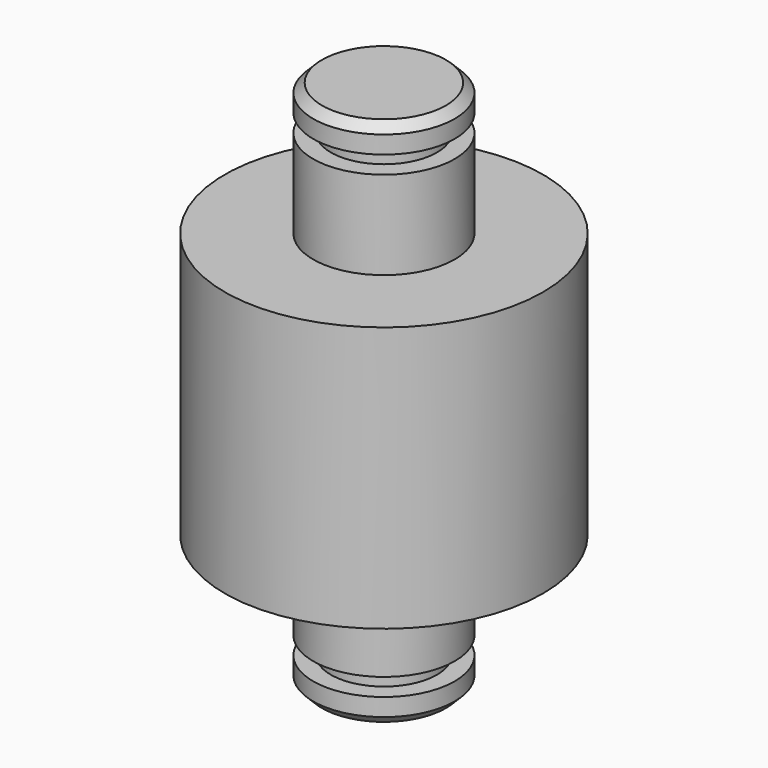
from build123d import *

# Parameters (mm, degrees)
F0_R     = 9
F1_DEPTH = 7.5
F2_R     = 4
F3_DEPTH = 7.5
F4_SIZE2 = 0.5
F4_SIZE  = 0.5
F5_W     = 1
F5_H     = 1


# Not quite as in the source:
# - a feature of the source that left no trace in its solid (it failed there, or was rolled back) is left out
# - a pattern or mirror of a feature is missing from the dataset's text; its kind, count and spacing are read off the source's solid


with BuildPart() as f1:
    # F0 (on Top) → F1 (new body, symmetric)
    with BuildSketch(Plane.XY):
        Circle(F0_R)
    extrude(amount=F1_DEPTH, both=True)

    # F2 (on face) → F3 (join)
    with BuildSketch(Plane.XY.offset(7.5)):
        Circle(F2_R)
    f3 = extrude(amount=F3_DEPTH)

    # F3_copies: F3 across plane
    add(f3.mirror(Plane(origin=(0, 0, 0), x_dir=(-1, 0, 0), z_dir=(0, 0, -1))))

    # F4
    f4_edges = [f1.edges().sort_by_distance(p)[0] for p in [
        (-4, 0, 15),
        (-4, 0, -15),
    ]]
    chamfer(f4_edges, length=F4_SIZE, length2=F4_SIZE2)

    # F5 (on Right) → F6 (revolve, cut)
    with BuildSketch(Plane.YZ):
        with Locations((3.5, 13)):
            Rectangle(F5_W, F5_H)
    f6 = revolve(axis=Axis((0, 0, 7.5), (0, 0, -1)), mode=Mode.SUBTRACT)

    # F6_copies: F6 across plane
    add(f6.mirror(Plane(origin=(0, 0, 0), x_dir=(-1, 0, 0), z_dir=(0, 0, -1))), mode=Mode.SUBTRACT)


solid = f1.part
